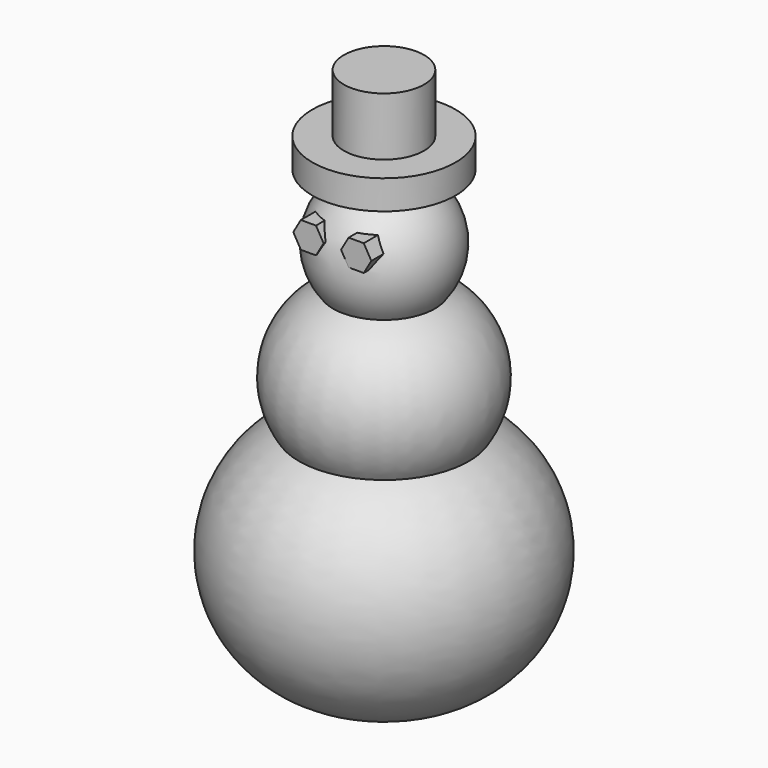
from build123d import *

# Parameters (mm, degrees)
F4_DEPTH = 6.604


with BuildPart() as f1:
    # F0 (on Front) → F1 (revolve)
    with BuildSketch(Plane.XZ):
        with BuildLine():
            ThreePointArc((-0.538991451, 54.1572621916), (-0.2695507401, 54.1654304357), (0, 54.1681535542))
            Line((0, 54.1681535542), (0, 71.5661346912))
            Line((0, 71.5661346912), (-8.1167221069, 71.5661346912))
            Line((-8.1167221069, 71.5661346912), (-8.1167221069, 59.7764104605))
            Line((-8.1167221069, 59.7764104605), (-14.5000517368, 59.7764104605))
            Line((-14.5000517368, 59.7764104605), (-14.5000517368, 53.8751520216))
            Line((-14.5000517368, 53.8751520216), (-0.538991451, 54.1572621916))
        make_face()
    revolve(axis=Axis((0, 0, 16.7530700564), (0, 0, -1)))


with BuildPart() as f1b:
    # F0 (on Front) → F1, piece 2 (revolve)
    with BuildSketch(Plane.XZ):
        with BuildLine():
            Line((0, 33.7650032795), (0, 54.1681535542))
            Line((0, 54.1681535542), (-0.538991451, 54.1572621916))
            ThreePointArc((-0.538991451, 54.1572621916), (-12.1783195865, 46.2760459099), (-10.3003703352, 32.345473914))
            ThreePointArc((-10.3003703352, 32.345473914), (-5.2604685043, 33.8554750958), (0, 33.7650032795))
        make_face()
    revolve(axis=Axis((0, 0, 16.7530700564), (0, 0, -1)))

    # F3 (on offset) → F4 (join)
    with BuildSketch(Plane.XZ.offset(6.35)):
        Polygon((-6.4620205134, 42.6593609154), (-3.397031042, 42.6593609154), (-1.8645363062, 45.31371966), (-3.397031042, 47.9680784047), (-6.4620205134, 47.9680784047), (-7.9945152492, 45.31371966), align=None)
        Polygon((3.2074333235, 42.6593609154), (6.272422795, 42.6593609154), (7.8049175307, 45.31371966), (6.272422795, 47.9680784047), (3.2074333235, 47.9680784047), (1.6749385878, 45.31371966), align=None)
    extrude(amount=F4_DEPTH)


with BuildPart() as f1c:
    # F0 (on Front) → F1, piece 3 (revolve)
    with BuildSketch(Plane.XZ):
        with BuildLine():
            ThreePointArc((0, 27.4836681783), (-5.6950589122, 28.7601848653), (-10.3003703352, 32.345473914))
            ThreePointArc((-10.3003703352, 32.345473914), (-19.4341830116, 21.4519730802), (-17.199848915, 7.4126481118))
            ThreePointArc((-17.199848915, 7.4126481118), (-8.8174635882, 10.174759831), (0, 9.7926855087))
            Line((0, 9.7926855087), (0, 27.4836681783))
        make_face()
    revolve(axis=Axis((0, 0, 16.7530700564), (0, 0, -1)))


with BuildPart() as f1d:
    # F0 (on Front) → F1, piece 4 (revolve)
    with BuildSketch(Plane.XZ):
        with BuildLine():
            ThreePointArc((0, 0), (-9.7024324023, 1.1481330031), (-17.199848915, 7.4126481118))
            ThreePointArc((-17.199848915, 7.4126481118), (-28.4067391947, -22.8155232955), (0, -38.0599945784))
            Line((0, -38.0599945784), (0, 0))
        make_face()
    revolve(axis=Axis((0, 0, 16.7530700564), (0, 0, -1)))


solid = Compound([f1.part, f1b.part, f1c.part, f1d.part])
